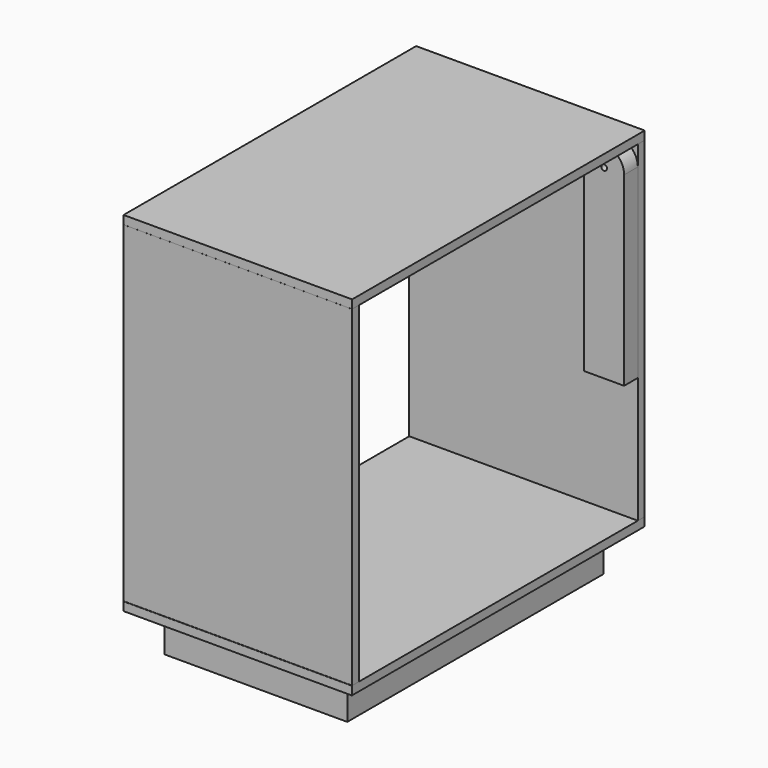
from build123d import *

# Parameters (mm, degrees)
F0_W      = 508
F0_H      = 736.6
F1_DEPTH  = 19.05
F4_W      = 508
F4_H      = 736.6
F5_DEPTH  = 19.05
F6_W      = 508
F6_H      = 812.8
F7_DEPTH  = 19.05
F8_W      = 508
F8_H      = 812.8
F9_DEPTH  = 19.05
F10_W     = 406.4
F10_H     = 711.8805297179
F10_W_2   = 330.2
F10_H_2   = 635.6805297179
F11_DEPTH = 88.9
F14_DEPTH = 38.1
F15_R     = 6.35
F16_DEPTH = 57.2386364558


with BuildPart() as f1:
    # F0 (on Front) → F1 (new body)
    with BuildSketch(Plane.XZ):
        with Locations((-254, -368.3)):
            Rectangle(F0_W, F0_H)
    extrude(amount=F1_DEPTH)


with BuildPart() as f5:
    # F4 (on offset) → F5 (new body)
    with BuildSketch(Plane(origin=(0, 793.75, 0), x_dir=(-1, 0, 0), z_dir=(0, 1, 0))):
        with Locations((254, -368.3)):
            Rectangle(F4_W, F4_H)
    extrude(amount=-F5_DEPTH)


with BuildPart() as f7:
    # F6 (on Top) → F7 (new body)
    with BuildSketch(Plane.XY):
        with Locations((-254, 387.4376364558)):
            Rectangle(F6_W, F6_H)
    extrude(amount=F7_DEPTH)


with BuildPart() as f9:
    # F8 (on offset) → F9 (new body)
    with BuildSketch(Plane.XY.offset(-755.65)):
        with Locations((-254, 386.6694702821)):
            Rectangle(F8_W, F8_H)
    extrude(amount=F9_DEPTH)

    # F10 (on offset) → F11 (join)
    with BuildSketch(Plane.XY.offset(-755.65)):
        with Locations((-254, 387.009735141)):
            Rectangle(F10_W, F10_H)
        with Locations((-254, 387.009735141)):
            Rectangle(F10_W_2, F10_H_2, mode=Mode.SUBTRACT)
    extrude(amount=-F11_DEPTH)


with BuildPart() as f14:
    # F13 (on offset) → F14 (new body)
    with BuildSketch(Plane.XZ.offset(-774.7)):
        with BuildLine():
            Line((-88.9, -457.2), (0, -457.2))
            Line((0, -457.2), (0, -44.45))
            ThreePointArc((0, -44.45), (-44.45, 0), (-88.9, -44.45))
            Line((-88.9, -44.45), (-88.9, -457.2))
        make_face()
    extrude(amount=F14_DEPTH)

    # F15 (on face) → F16 (cut, through all)
    with BuildSketch(Plane.XZ.offset(-736.6)):
        with Locations((-44.45, -44.45)):
            Circle(F15_R)
    extrude(amount=-F16_DEPTH, mode=Mode.SUBTRACT)


solid = Compound([f1.part, f5.part, f7.part, f9.part, f14.part])
